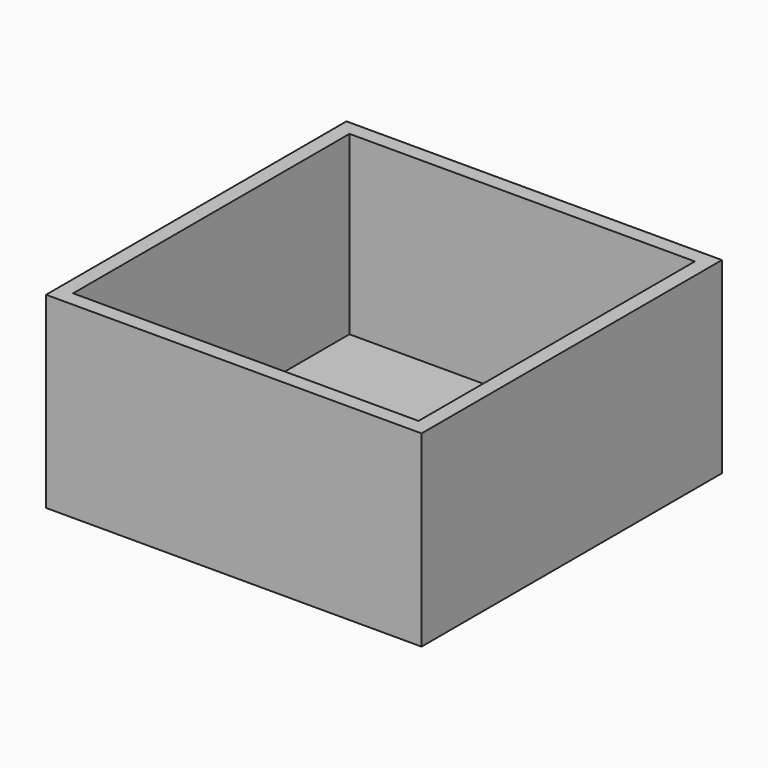
from build123d import *

# Parameters (mm, degrees)
F0_W         = 20
F0_H         = 20
F0_W_2       = 18.4
F0_H_2       = 18.4
F1_DEPTH     = 10
F2_DEPTH     = 0.6
F3_TEXT_SIZE = 18.6741410289
F4_DEPTH     = 0.2


# Not quite as in the source:
# - Text() gives the source's letters only with a copy of the font that has no kerning and outlines rounded to 1/6400 em; it was checked with that copy


with BuildPart() as f1:
    # F0 (on Top) → F1 (new body)
    with BuildSketch(Plane.XY):
        Rectangle(F0_W, F0_H)
        Rectangle(F0_W_2, F0_H_2, mode=Mode.SUBTRACT)
    extrude(amount=F1_DEPTH)

    # F0 (on Top) → F2 (join)
    with BuildSketch(Plane.XY):
        Rectangle(F0_W, F0_H)
        Rectangle(F0_W_2, F0_H_2, mode=Mode.SUBTRACT)
        Rectangle(F0_W_2, F0_H_2)
    extrude(amount=F2_DEPTH)

    # F3 (on face) → F4 (cut)
    with BuildSketch(Plane.XY.offset(0.6)):
        with Locations((-5.974045489, -6.3751991838)):
            Text('4', F3_TEXT_SIZE, font='Open Sans', font_style=FontStyle.BOLD, text_align=(TextAlign.LEFT, TextAlign.BOTTOM))
    extrude(amount=-F4_DEPTH, mode=Mode.SUBTRACT)


solid = f1.part
